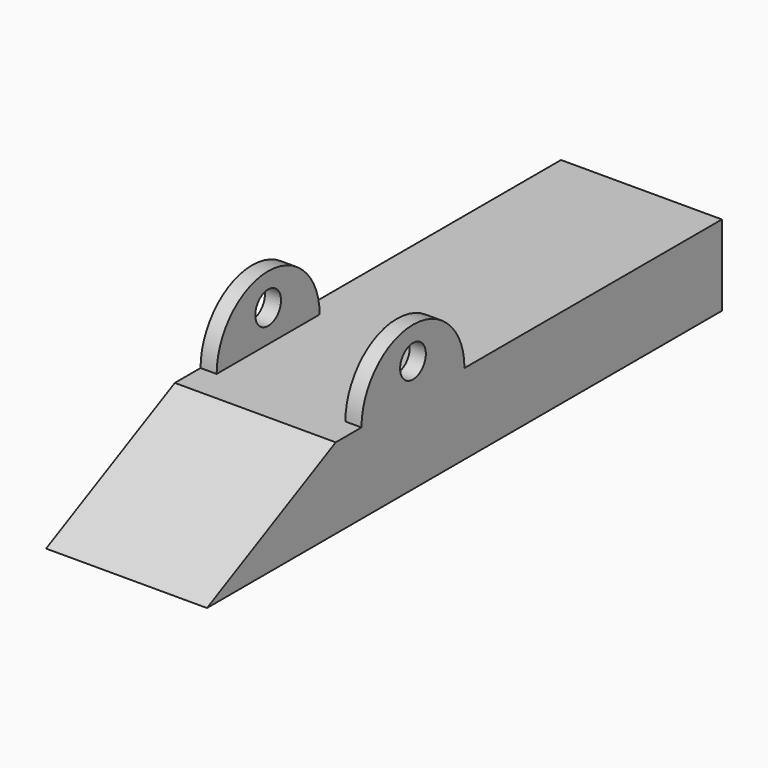
from build123d import *

# Parameters (mm, degrees)
F0_W     = 10
F0_H     = 5
F1_DEPTH = 40
F2_R     = 1
F3_DEPTH = 1
F4_R     = 1
F5_DEPTH = 1
F6_SIZE2 = 4.99999
F6_SIZE  = 9.99999


# Not quite as in the source:
# - a fillet or chamfer is up to 0.001 mm smaller than in the source, because OpenCascade refuses the exact size


with BuildPart() as f1:
    # F0 (on Front) → F1 (new body)
    with BuildSketch(Plane.XZ):
        Rectangle(F0_W, F0_H)
    extrude(amount=F1_DEPTH)

    # F2 (on face) → F3 (join)
    with BuildSketch(Plane.YZ.offset(5)):
        with BuildLine():
            Line((-24, 2.5), (-20, 2.5))
            ThreePointArc((-20, 2.5), (-24, 6.5), (-28, 2.5))
            Line((-28, 2.5), (-24, 2.5))
        make_face()
        with Locations((-24, 4.5)):
            Circle(F2_R, mode=Mode.SUBTRACT)
    extrude(amount=-F3_DEPTH)

    # F4 (on face) → F5 (join)
    with BuildSketch(Plane(origin=(-5, 0, 0), x_dir=(0, -1, 0), z_dir=(-1, 0, 0))):
        with BuildLine():
            ThreePointArc((28, 2.5), (24, 6.5), (20, 2.5))
            Line((20, 2.5), (24, 2.5))
            Line((24, 2.5), (28, 2.5))
        make_face()
        with Locations((24, 4.5)):
            Circle(F4_R, mode=Mode.SUBTRACT)
    extrude(amount=-F5_DEPTH)

    # F6 (size 10 and 5 in the source; OpenCascade refuses exactly that, so slightly less here)
    f6_edges = [f1.edges().sort_by_distance(p)[0] for p in [
        (0, -40, 2.5),
    ]]
    f6_side = f1.faces().sort_by_distance((0, -19.833333, 2.5))[0]
    chamfer(f6_edges, length=F6_SIZE, length2=F6_SIZE2, reference=f6_side)


solid = f1.part
